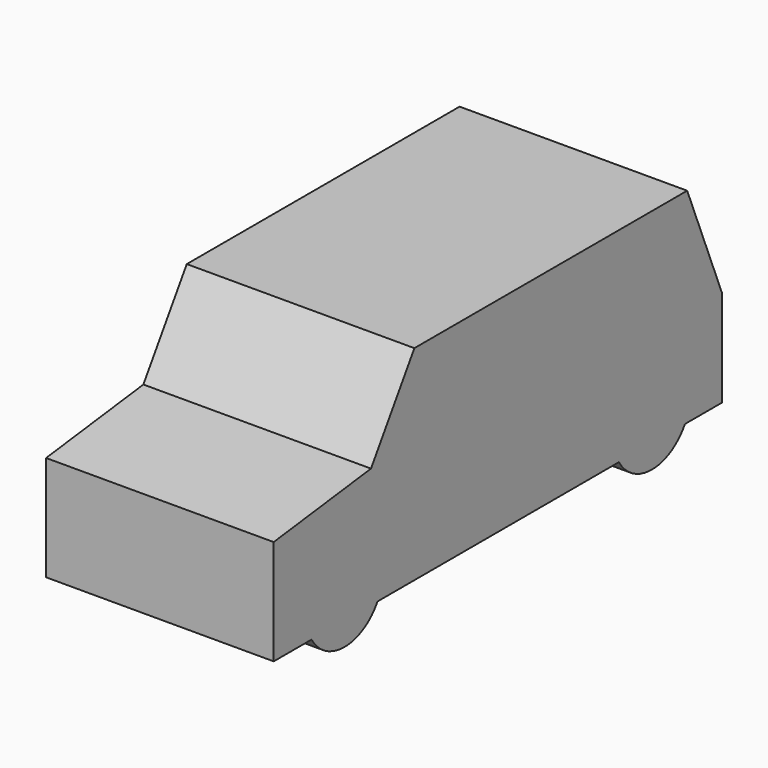
from build123d import *

# Parameters (mm, degrees)
F0_W     = 1981.2
F0_H     = 4876.8
F1_DEPTH = 3048
F3_DEPTH = 6096


with BuildPart() as f1:
    # F0 (on Top) → F1 (new body)
    with BuildSketch(Plane.XY):
        Rectangle(F0_W, F0_H)
    extrude(amount=F1_DEPTH)

    # F2 (on face) → F3 (cut)
    with BuildSketch(Plane(origin=(-990.6, 0, 0), x_dir=(0, -1, 0), z_dir=(-1, 0, 0))):
        Polygon((1379.873641154, 1250.2053831043), (2438.4, 1117.6), (2438.4, 3048), (-2438.4, 3048), (-2438.4, 1045.6442832947), (-2060.410954721, 1981.2), (907.7037284231, 1981.2), align=None)
        with BuildLine():
            Line((2438.4, 0), (2438.4, 203.2))
            Line((2438.4, 203.2), (2027.0615872515, 203.2))
            ThreePointArc((2027.0615872515, 203.2), (1874.2019202661, 54.320273291), (1667.8513478767, 0))
            Line((1667.8513478767, 0), (2438.4, 0))
        make_face()
        with BuildLine():
            ThreePointArc((1667.8513478767, 0), (1461.5007693106, 54.3202705987), (1308.641097566, 203.2))
            Line((1308.641097566, 203.2), (-1317.311745224, 203.2))
            ThreePointArc((-1317.311745224, 203.2), (-1470.171414589, 54.3202719448), (-1676.5219900668, 0))
            Line((-1676.5219900668, 0), (1667.8513478767, 0))
        make_face()
        with BuildLine():
            Line((-2438.4, 0), (-1676.5219900668, 0))
            ThreePointArc((-1676.5219900668, 0), (-1882.8725655446, 54.3202719448), (-2035.7322349096, 203.2))
            Line((-2035.7322349096, 203.2), (-2438.4, 203.2))
            Line((-2438.4, 203.2), (-2438.4, 0))
        make_face()
    extrude(amount=-F3_DEPTH, mode=Mode.SUBTRACT)


solid = f1.part
